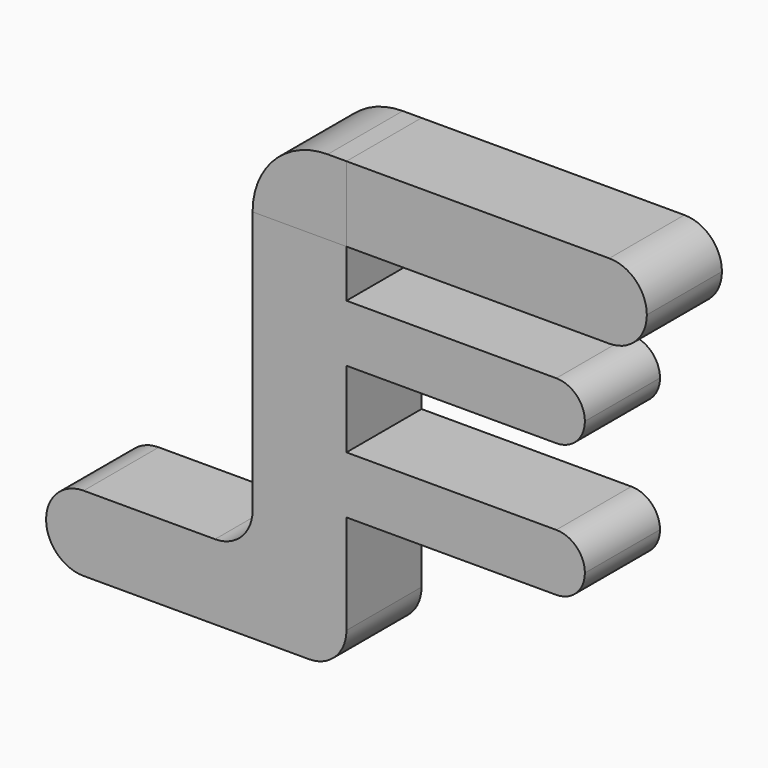
from build123d import *

# Parameters (mm, degrees)
F0_W      = 2.5
F0_H      = 2.5
F1_DEPTH  = 10
F2_W      = 2.5
F2_H      = 2
F3_DEPTH  = 8
F4_W      = 2.5
F4_H      = 2
F5_DEPTH  = 2.5
F6_W      = 8
F6_H      = 2.5
F7_DEPTH  = 2
F8_R      = 0.99999
F9_W      = 2.5
F9_H      = 2.5
F10_DEPTH = 2
F11_R     = 1.99999
F12_W     = 2.5
F12_H     = 5.08
F13_DEPTH = 6.35
F14_W     = 6.35
F14_H     = 2.032
F15_DEPTH = 2.501
F16_R     = 0.76199


# Not quite as in the source:
# - a fillet or chamfer is up to 0.001 mm smaller than in the source, because OpenCascade refuses the exact size


with BuildPart() as f1:
    # F0 (on Top) → F1 (new body)
    with BuildSketch(Plane.XY):
        with Locations((-19.965537297, -2.8490219265)):
            Rectangle(F0_W, F0_H)
    extrude(amount=F1_DEPTH)

    # F2 (on face) → F3 (join)
    with BuildSketch(Plane.YZ.offset(-18.715537297)):
        with Locations((-2.8490219265, 9)):
            Rectangle(F2_W, F2_H)
    extrude(amount=F3_DEPTH)

    # F4 (on face) → F5 (cut, through all)
    with BuildSketch(Plane.XZ.offset(4.0990219265)):
        with Locations((-19.965537297, 9)):
            Rectangle(F4_W, F4_H)
    extrude(amount=-F5_DEPTH, mode=Mode.SUBTRACT)

    # F6 (on face) → F7 (join)
    with BuildSketch(Plane(origin=(0, 0, 0), x_dir=(1, 0, 0), z_dir=(0, 0, -1))):
        with Locations((-22.715537297, 2.8490219265)):
            Rectangle(F6_W, F6_H)
    extrude(amount=F7_DEPTH)

    # F8 (radius 1 in the source; OpenCascade refuses exactly that, so slightly less here)
    f8_edges = [f1.edges().sort_by_distance(p)[0] for p in [
        (-21.215537, -2.849022, 0),
        (-26.715537, -2.849022, 0),
        (-10.715537, -2.849022, 10),
        (-10.715537, -2.849022, 8),
        (-18.715537, -2.849022, -2),
        (-26.715537, -2.849022, -2),
    ]]
    fillet(f8_edges, radius=F8_R)

    # F12 (on face) → F13 (join)
    with BuildSketch(Plane.YZ.offset(-18.715537297)):
        with Locations((-2.8490219265, 4.19)):
            Rectangle(F12_W, F12_H)
    extrude(amount=F13_DEPTH)

    # F14 (on face) → F15 (cut, through all)
    with BuildSketch(Plane.XZ.offset(4.0990219265)):
        with Locations((-15.540537297, 4.19)):
            Rectangle(F14_W, F14_H)
    extrude(amount=-F15_DEPTH, mode=Mode.SUBTRACT)

    # F16 (radius 0.762 in the source; OpenCascade refuses exactly that, so slightly less here)
    f16_edges = [f1.edges().sort_by_distance(p)[0] for p in [
        (-12.365537, -2.849022, 6.73),
        (-12.365537, -2.849022, 5.206),
        (-12.365537, -2.849022, 3.174),
        (-12.365537, -2.849022, 1.65),
    ]]
    fillet(f16_edges, radius=F16_R)


with BuildPart() as f10:
    # F9 (on face) → F10 (new body, through all)
    with BuildSketch(Plane.XY.offset(8)):
        with Locations((-19.965537297, -2.8490219265)):
            Rectangle(F9_W, F9_H)
    extrude(amount=F10_DEPTH)

    # F11 (radius 2 in the source; OpenCascade refuses exactly that, so slightly less here)
    f11_edges = [f10.edges().sort_by_distance(p)[0] for p in [
        (-21.215537, -2.849022, 10),
    ]]
    fillet(f11_edges, radius=F11_R)


solid = Compound([f1.part, f10.part])
